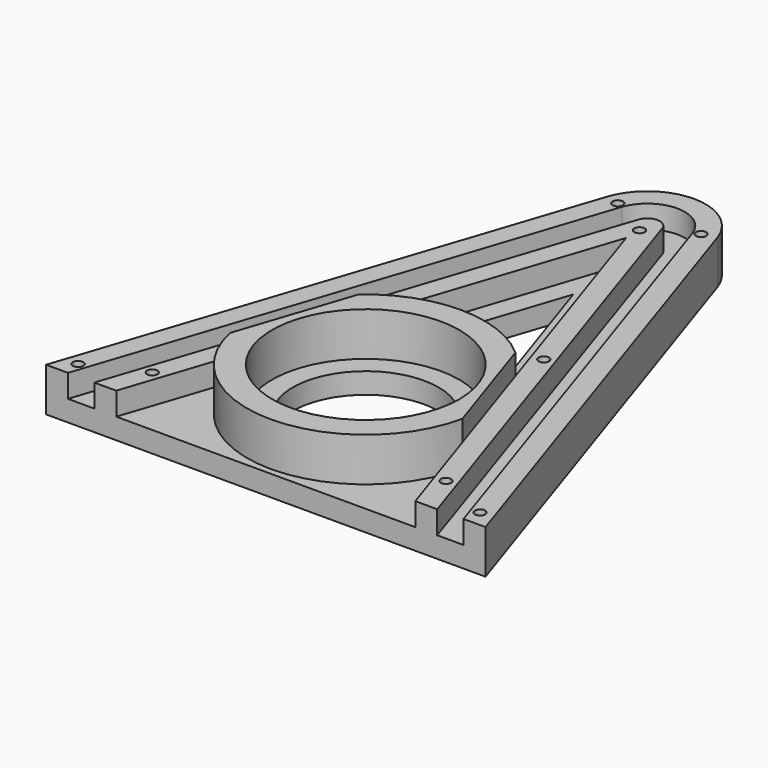
from build123d import *

# Parameters (mm, degrees)
F1_DEPTH  = 5
F3_DEPTH  = 5.5
F5_DEPTH  = 5.5
F6_R      = 22.5
F7_DEPTH  = 10.5
F8_R      = 17.5
F9_DEPTH  = 25
F11_DEPTH = 25
F12_R     = 1.25
F13_DEPTH = 11
F14_R     = 2.25
F15_DEPTH = 2.5


with BuildPart() as f1:
    # F0 (on Top) → F1 (new body)
    with BuildSketch(Plane.XY):
        with BuildLine():
            Line((50.7170443075, -14.5414772037), (55.9852813742, -14.5414772037))
            Line((55.9852813742, -14.5414772037), (16.9705627485, 103))
            ThreePointArc((16.9705627485, 103), (8.4852813742, 109), (0, 103))
            Line((0, 103), (-39.0147186258, -14.5414772037))
            Line((-39.0147186258, -14.5414772037), (-33.746481559, -14.5414772037))
            Line((-33.746481559, -14.5414772037), (4.7271265323, 101.3697708508))
            ThreePointArc((4.7271265323, 101.3697708508), (8.4852813742, 104), (12.2434362162, 101.3697708508))
            Line((12.2434362162, 101.3697708508), (50.7170443075, -14.5414772037))
        make_face()
        with BuildLine():
            Line((16.9705627485, 103), (55.9852813742, -14.5414772037))
            Line((55.9852813742, -14.5414772037), (61.253518441, -14.5414772037))
            Line((61.253518441, -14.5414772037), (21.7024158273, 104.6159892602))
            ThreePointArc((21.7024158273, 104.6159892602), (8.4852813742, 114), (-4.7318530788, 104.6159892602))
            Line((-4.7318530788, 104.6159892602), (-44.2829556925, -14.5414772037))
            Line((-44.2829556925, -14.5414772037), (-39.0147186258, -14.5414772037))
            Line((-39.0147186258, -14.5414772037), (0, 103))
            ThreePointArc((0, 103), (8.4852813742, 109), (16.9705627485, 103))
        make_face()
        with BuildLine():
            Line((-33.746481559, -14.5414772037), (50.7170443075, -14.5414772037))
            Line((50.7170443075, -14.5414772037), (12.2434362162, 101.3697708508))
            ThreePointArc((12.2434362162, 101.3697708508), (8.4852813742, 104), (4.7271265323, 101.3697708508))
            Line((4.7271265323, 101.3697708508), (-33.746481559, -14.5414772037))
        make_face()
    extrude(amount=F1_DEPTH)

    # F2 (on face) → F3 (join)
    with BuildSketch(Plane.XY.offset(5)):
        with BuildLine():
            Line((-39.0147186258, -14.5414772037), (0, 103))
            ThreePointArc((0, 103), (8.4852813742, 109), (16.9705627485, 103))
            Line((16.9705627485, 103), (55.9852813742, -14.5414772037))
            Line((55.9852813742, -14.5414772037), (61.253518441, -14.5414772037))
            Line((61.253518441, -14.5414772037), (21.7024158273, 104.6159892602))
            ThreePointArc((21.7024158273, 104.6159892602), (8.4852813742, 114), (-4.7318530788, 104.6159892602))
            Line((-4.7318530788, 104.6159892602), (-44.2829556925, -14.5414772037))
            Line((-44.2829556925, -14.5414772037), (-39.0147186258, -14.5414772037))
        make_face()
    extrude(amount=F3_DEPTH)

    # F4 (on face) → F5 (join)
    with BuildSketch(Plane.XY.offset(5)):
        with BuildLine():
            ThreePointArc((11.29925422, 101.0399792418), (8.4852813742, 103), (5.6713085285, 101.0399792418))
            Line((5.6713085285, 101.0399792418), (-32.6928341457, -14.5414772037))
            Line((-32.6928341457, -14.5414772037), (-27.424597079, -14.5414772037))
            Line((-27.424597079, -14.5414772037), (8.4852813742, 93.6459020283))
            Line((8.4852813742, 93.6459020283), (44.3951598274, -14.5414772037))
            Line((44.3951598274, -14.5414772037), (49.6633968942, -14.5414772037))
            Line((49.6633968942, -14.5414772037), (11.29925422, 101.0399792418))
        make_face()
    extrude(amount=F5_DEPTH)

    # F6 (on face) → F7 (join)
    with BuildSketch(Plane.XY.offset(5)):
        with BuildLine():
            Line((36.3787330735, 9.6099885954), (27.3452487141, 36.8255916626))
            ThreePointArc((27.3452487141, 36.8255916626), (8.4852813742, 43.9585227963), (-10.3746859657, 36.8255916626))
            Line((-10.3746859657, 36.8255916626), (-19.4081703251, 9.6099885954))
            ThreePointArc((-19.4081703251, 9.6099885954), (8.4852813742, -13.0414772037), (36.3787330735, 9.6099885954))
        make_face()
        with Locations((8.4852813742, 15.4585227963)):
            Circle(F6_R, mode=Mode.SUBTRACT)
    extrude(amount=F7_DEPTH)

    # F8 (on face) → F9 (cut)
    with BuildSketch(Plane.XY.offset(5)):
        with Locations((8.4852813742, 15.4585227963)):
            Circle(F8_R)
    extrude(amount=-F9_DEPTH, mode=Mode.SUBTRACT)

    # F10 (on face) → F11 (cut)
    with BuildSketch(Plane.XY.offset(5)):
        with BuildLine():
            Line((8.4852813742, 77.7740365146), (-1.5945371695, 47.4060932537))
            ThreePointArc((-1.5945371695, 47.4060932537), (8.4852813742, 48.9585227963), (18.5650999179, 47.4060932537))
            Line((18.5650999179, 47.4060932537), (8.4852813742, 77.7740365146))
        make_face()
    extrude(amount=-F11_DEPTH, mode=Mode.SUBTRACT)

    # F12 (on face) → F13 (cut)
    with BuildSketch(Plane.XY.offset(10.5)):
        with Locations((8.4959140697, 97.6459020283)):
            Circle(F12_R)
        with Locations((-1.5147186258, 103.6459020283)):
            Circle(F12_R)
        with Locations((18.4852813742, 103.6459020283)):
            Circle(F12_R)
        with Locations((-10.2829556925, 45.4585227963)):
            Circle(F12_R)
        with Locations((27.253518441, 45.4585227963)):
            Circle(F12_R)
        with Locations((56.753518441, -10.5414772037)):
            Circle(F12_R)
        with Locations((43.753518441, -4.5414772037)):
            Circle(F12_R)
        with Locations((-26.7829556925, -4.5414772037)):
            Circle(F12_R)
        with Locations((-39.7829556925, -10.5414772037)):
            Circle(F12_R)
    extrude(amount=-F13_DEPTH, mode=Mode.SUBTRACT)

    # F14 (on face) → F15 (cut)
    with BuildSketch(Plane(origin=(0, 0, 0), x_dir=(1, 0, 0), z_dir=(0, 0, -1))):
        with Locations((18.4852813742, -103.6459020283)):
            Circle(F14_R)
        with Locations((8.4959140697, -97.6459020283)):
            Circle(F14_R)
        with Locations((-1.5147186258, -103.6459020283)):
            Circle(F14_R)
        with Locations((-10.2829556925, -45.4585227963)):
            Circle(F14_R)
        with Locations((27.253518441, -45.4585227963)):
            Circle(F14_R)
        with Locations((-39.7829556925, 10.5414772037)):
            Circle(F14_R)
        with Locations((-26.7829556925, 4.5414772037)):
            Circle(F14_R)
        with Locations((43.753518441, 4.5414772037)):
            Circle(F14_R)
        with Locations((56.753518441, 10.5414772037)):
            Circle(F14_R)
    extrude(amount=-F15_DEPTH, mode=Mode.SUBTRACT)


solid = f1.part
